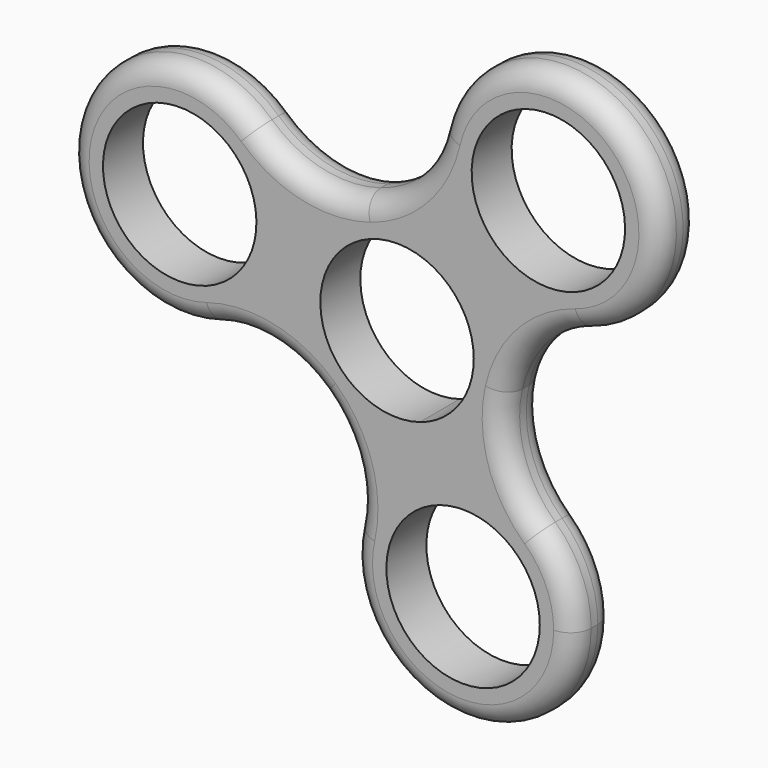
from build123d import *

# Parameters (mm, degrees)
F1_DEPTH = 7.2
F2_R     = 3


# Not quite as in the source:
# - ends of sketch curves that miss each other by under 0.0002 mm in the source are joined


with BuildPart() as f1:
    # F0 (on Front) → F1 (new body)
    with BuildSketch(Plane.XZ):
        with BuildLine():
            ThreePointArc((-26.551024914, -8.237140674), (-19.523549824, -3.8055536516), (-15.6533710357, 3.546050651))
            ThreePointArc((-15.6533710357, 3.546050651), (-15.3562075484, 5.3080195325), (-15.256742113, 7.0921011182))
            ThreePointArc((-15.256742113, 7.0921011182), (-16.6011328418, 13.5223076439), (-20.4090855352, 18.875291735))
            ThreePointArc((-20.4090855352, 18.875291735), (-46.9601131695, 10.6381516773), (-26.551024914, -8.237140674))
        make_face()
        with BuildLine():
            ThreePointArc((-20.256742113, 7.0921011182), (-20.3252214351, 5.8638081562), (-20.529810638, 4.6507392068))
            ThreePointArc((-20.529810638, 4.6507392068), (-42.2882627909, 8.3203940802), (-20.256742113, 7.0921011182))
        make_face(mode=Mode.SUBTRACT)
        with BuildLine():
            ThreePointArc((-15.256742113, 7.0921011182), (-15.3562075484, 5.3080195325), (-15.6533710357, 3.546050651))
            ThreePointArc((-15.6533710357, 3.546050651), (-11.7831915214, 10.8976555997), (-4.7557152197, 15.3292424062))
            ThreePointArc((-4.7557152197, 15.3292424062), (-13.0574808704, 15.0051132532), (-20.4090855352, 18.875291735))
            ThreePointArc((-20.4090855352, 18.875291735), (-16.6011328418, 13.5223076439), (-15.256742113, 7.0921011182))
        make_face()
        with BuildLine():
            ThreePointArc((-4.7557152197, 15.3292424062), (3.5460508162, 15.6533709983), (10.8976554434, 11.783191666))
            ThreePointArc((10.8976554434, 11.783191666), (6.46606877, 18.8106669593), (6.1419393788, 27.112432409))
            ThreePointArc((6.1419393788, 27.112432409), (2.2717599984, 19.7608287216), (-4.7557152197, 15.3292424062))
        make_face()
        with BuildLine():
            ThreePointArc((-10.776931475, 2.4413619114), (-3.2741843024, 10.5537773879), (7.5027471726, 8.1124154765))
            Line((7.5027471726, 8.1124154765), (10.8976553955, 11.7831917102))
            ThreePointArc((10.8976554434, 11.783191666), (3.5460508162, 15.6533709983), (-4.7557152197, 15.3292424062))
            ThreePointArc((-4.7557152197, 15.3292424062), (-11.7831915214, 10.8976555997), (-15.6533710357, 3.546050651))
            Line((-15.6533710565, 3.5460505591), (-10.776931475, 2.4413619114))
        make_face()
        with BuildLine():
            ThreePointArc((6.1419393788, 27.112432409), (6.46606877, 18.8106669593), (10.8976554434, 11.783191666))
            ThreePointArc((10.8976554434, 11.783191666), (18.2492594785, 7.9130125347), (26.551024914, 8.237140674))
            ThreePointArc((26.551024914, 8.237140674), (34.7168376295, 14.0460554763), (37.8453107911, 23.5663834205))
            ThreePointArc((37.8453107911, 23.5663834205), (23.5793916234, 39.5169180693), (6.1419393788, 27.112432409))
        make_face()
        with BuildLine():
            ThreePointArc((32.8453107911, 23.5663834205), (26.2223382217, 13.4419610602), (14.2925636184, 15.453967944))
            ThreePointArc((14.2925636184, 15.453967944), (17.3682833605, 33.6908057807), (32.8453107911, 23.5663834205))
        make_face(mode=Mode.SUBTRACT)
        with BuildLine():
            ThreePointArc((26.551024914, 8.237140674), (18.2492594785, 7.9130125347), (10.8976554434, 11.783191666))
            ThreePointArc((10.8976554434, 11.783191666), (14.7056089617, 6.4302072336), (16.05, 0))
            ThreePointArc((16.05, 0), (15.9505345891, -1.7840813666), (15.6533711747, -3.5460500371))
            ThreePointArc((15.6533711747, -3.5460500371), (19.5235500377, 3.8055538826), (26.551024914, 8.237140674))
        make_face()
        with BuildLine():
            ThreePointArc((15.6533711747, -3.5460500371), (11.7831918467, -10.8976552479), (4.7557155338, -15.3292423088))
            ThreePointArc((4.7557155338, -15.3292423088), (13.0574810308, -15.0051132896), (20.4090855352, -18.875291735))
            ThreePointArc((20.4090855352, -18.875291735), (15.9774995258, -11.8478157546), (15.6533711747, -3.5460500371))
        make_face()
        with BuildLine():
            ThreePointArc((7.5027471726, 8.1124154765), (10.1244223603, 4.4270274306), (11.05, 0))
            ThreePointArc((11.05, 0), (8.8961293983, -6.5544932473), (3.2741843024, -10.5537773879))
            Line((3.2741843024, -10.5537773879), (4.755715661, -15.3292422693))
            ThreePointArc((4.755715661, -15.3292422693), (11.7831918467, -10.8976552479), (15.6533711747, -3.5460500371))
            ThreePointArc((15.6533711747, -3.5460500371), (15.9505345891, -1.7840813666), (16.05, 0))
            ThreePointArc((16.05, 0), (14.7056089617, 6.4302072336), (10.8976554434, 11.783191666))
            Line((10.8976554434, 11.783191666), (7.5027471726, 8.1124154765))
        make_face()
        with BuildLine():
            Line((4.755715661, -15.3292422693), (3.2741843024, -10.5537773879))
            ThreePointArc((3.2741843024, -10.5537773879), (-7.5027471726, -8.1124154765), (-10.776931475, 2.4413619114))
            Line((-10.776931475, 2.4413619114), (-15.6533710565, 3.5460505591))
            ThreePointArc((-15.6533710565, 3.5460505591), (-15.3292423483, -4.7557154063), (-10.8976557178, -11.7831914121))
            ThreePointArc((-10.8976557178, -11.7831914121), (-3.5460508381, -15.6533709933), (4.755715661, -15.3292422693))
        make_face()
        with BuildLine():
            ThreePointArc((-10.8976557178, -11.7831914121), (-15.3292423483, -4.7557154063), (-15.6533710357, 3.546050651))
            ThreePointArc((-15.6533710357, 3.546050651), (-19.523549824, -3.8055536516), (-26.551024914, -8.237140674))
            ThreePointArc((-26.551024914, -8.237140674), (-18.2492596608, -7.9130124934), (-10.8976557178, -11.7831914121))
        make_face()
        with BuildLine():
            ThreePointArc((-6.1419393788, -27.112432409), (-2.2717598868, -19.7608286009), (4.7557155338, -15.3292423088))
            ThreePointArc((4.7557155338, -15.3292423088), (-3.5460508381, -15.6533709933), (-10.8976557178, -11.7831914121))
            ThreePointArc((-10.8976557178, -11.7831914121), (-6.4660688254, -18.8106667808), (-6.1419393788, -27.112432409))
        make_face()
        with BuildLine():
            ThreePointArc((20.4090855352, -18.875291735), (13.0574810308, -15.0051132896), (4.7557155338, -15.3292423088))
            ThreePointArc((4.7557155338, -15.3292423088), (-2.2717598868, -19.7608286009), (-6.1419393788, -27.112432409))
            ThreePointArc((-6.1419393788, -27.112432409), (7.7273488892, -46.6090190085), (25.5614313219, -30.6584845387))
            ThreePointArc((25.5614313219, -30.6584845387), (24.2170399479, -24.2282765375), (20.4090855352, -18.875291735))
        make_face()
        with BuildLine():
            ThreePointArc((20.5614313219, -30.6584845387), (2.9569380746, -39.5546139369), (6.2372470195, -20.1047071508))
            ThreePointArc((6.2372470195, -20.1047071508), (16.0659245692, -21.7623551404), (20.5614313219, -30.6584845387))
        make_face(mode=Mode.SUBTRACT)
    extrude(amount=-F1_DEPTH)

    # F2
    f2_edges = [f1.edges().sort_by_distance(p)[0] for p in [
        (-4.755716, 0, 15.329242),
        (-10.897655, 7.2, -11.783192),
    ]]
    fillet(f2_edges, radius=F2_R)


solid = f1.part
